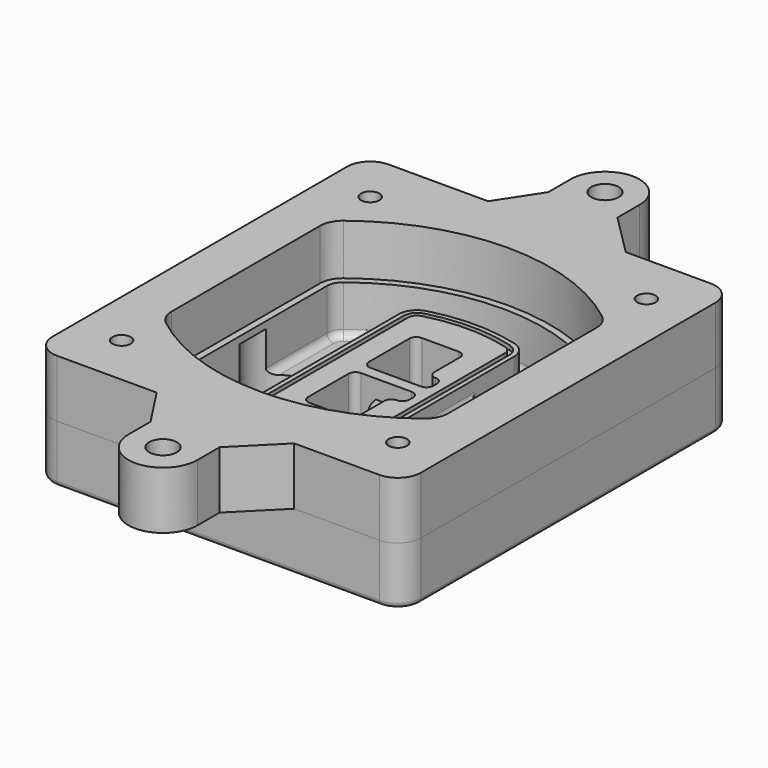
from build123d import *

# Parameters (mm, degrees)
F0_R      = 4
F1_DEPTH  = 25
F2_DEPTH  = 3
F3_DEPTH  = 18
F5_DEPTH  = 21
F6_DEPTH  = 2
F8_DEPTH  = 20
F9_DEPTH  = 16
F10_DEPTH = 25
F7_R      = 6
F7_R_2    = 4
F11_DEPTH = 6
F13_DEPTH = 9
F14_R     = 3
F15_R     = 2
F16_R     = 4
F16_R_2   = 6
F17_DEPTH = 25
F18_DEPTH = 25


# Not quite as in the source:
# - a feature names something its author has since deleted; it is built from what else it names


with BuildPart() as f1:
    # F0 (on Top) → F1 (new body)
    with BuildSketch(Plane.XY):
        with BuildLine():
            ThreePointArc((-80, -80), (-77.0710678119, -87.0710678119), (-70, -90))
            Line((-70, -90), (70, -90))
            ThreePointArc((70, -90), (77.0710678119, -87.0710678119), (80, -80))
            Line((80, -80), (80, 80))
            ThreePointArc((80, 80), (77.0710678119, 87.0710678119), (70, 90))
            Line((70, 90), (-70, 90))
            ThreePointArc((-70, 90), (-77.0710678119, 87.0710678119), (-80, 80))
            Line((-80, 80), (-80, -80))
        make_face()
        with Locations((-60, -67.5)):
            Circle(F0_R, mode=Mode.SUBTRACT)
        with Locations((60, -67.5)):
            Circle(F0_R, mode=Mode.SUBTRACT)
        with Locations((-60, 67.5)):
            Circle(F0_R, mode=Mode.SUBTRACT)
        with BuildLine():
            ThreePointArc((-64, 40.2934422872), (-62.5820384798, 46.4328484224), (-58.6153846154, 51.3286200352))
            ThreePointArc((-58.6153846154, 51.3286200352), (0, 71.5), (58.6153846154, 51.3286200352))
            ThreePointArc((58.6153846154, 51.3286200352), (62.5820384798, 46.4328484224), (64, 40.2934422872))
            Line((64, 40.2934422872), (64, -40.2934422872))
            ThreePointArc((64, -40.2934422872), (62.5820384798, -46.4328484224), (58.6153846154, -51.3286200352))
            ThreePointArc((58.6153846154, -51.3286200352), (0, -71.5), (-58.6153846154, -51.3286200352))
            ThreePointArc((-58.6153846154, -51.3286200352), (-62.5820384798, -46.4328484224), (-64, -40.2934422872))
            Line((-64, -40.2934422872), (-64, 40.2934422872))
        make_face(mode=Mode.SUBTRACT)
        with Locations((60, 67.5)):
            Circle(F0_R, mode=Mode.SUBTRACT)
        with BuildLine():
            ThreePointArc((58.6153846154, 51.3286200352), (0, 71.5), (-58.6153846154, 51.3286200352))
            ThreePointArc((-58.6153846154, 51.3286200352), (-62.5820384798, 46.4328484224), (-64, 40.2934422872))
            Line((-64, 40.2934422872), (-64, -40.2934422872))
            ThreePointArc((-64, -40.2934422872), (-62.5820384798, -46.4328484224), (-58.6153846154, -51.3286200352))
            ThreePointArc((-58.6153846154, -51.3286200352), (0, -71.5), (58.6153846154, -51.3286200352))
            ThreePointArc((58.6153846154, -51.3286200352), (62.5820384798, -46.4328484224), (64, -40.2934422872))
            Line((64, -40.2934422872), (64, 40.2934422872))
            ThreePointArc((64, 40.2934422872), (62.5820384798, 46.4328484224), (58.6153846154, 51.3286200352))
        make_face()
        with BuildLine():
            Line((-60, -40.2934422872), (-60, 40.2934422872))
            ThreePointArc((-60, 40.2934422872), (-58.9871703427, 44.6787323838), (-56.1538461538, 48.1757121072))
            ThreePointArc((-56.1538461538, 48.1757121072), (0, 67.5), (56.1538461538, 48.1757121072))
            ThreePointArc((56.1538461538, 48.1757121072), (58.9871703427, 44.6787323838), (60, 40.2934422872))
            Line((60, 40.2934422872), (60, -40.2934422872))
            ThreePointArc((60, -40.2934422872), (58.9871703427, -44.6787323838), (56.1538461538, -48.1757121072))
            ThreePointArc((56.1538461538, -48.1757121072), (0, -67.5), (-56.1538461538, -48.1757121072))
            ThreePointArc((-56.1538461538, -48.1757121072), (-58.9871703427, -44.6787323838), (-60, -40.2934422872))
        make_face(mode=Mode.SUBTRACT)
        with BuildLine():
            ThreePointArc((-56.1538461538, 48.1757121072), (-58.9871703427, 44.6787323838), (-60, 40.2934422872))
            Line((-60, 40.2934422872), (-60, -40.2934422872))
            ThreePointArc((-60, -40.2934422872), (-58.9871703427, -44.6787323838), (-56.1538461538, -48.1757121072))
            ThreePointArc((-56.1538461538, -48.1757121072), (0, -67.5), (56.1538461538, -48.1757121072))
            ThreePointArc((56.1538461538, -48.1757121072), (58.9871703427, -44.6787323838), (60, -40.2934422872))
            Line((60, -40.2934422872), (60, 40.2934422872))
            ThreePointArc((60, 40.2934422872), (58.9871703427, 44.6787323838), (56.1538461538, 48.1757121072))
            ThreePointArc((56.1538461538, 48.1757121072), (0, 67.5), (-56.1538461538, 48.1757121072))
        make_face()
        with BuildLine():
            ThreePointArc((54.3076923077, 45.8110311612), (56.2910192399, 43.3631453548), (57, 40.2934422872))
            Line((57, 40.2934422872), (57, -40.2934422872))
            ThreePointArc((57, -40.2934422872), (56.2910192399, -43.3631453548), (54.3076923077, -45.8110311612))
            ThreePointArc((54.3076923077, -45.8110311612), (0, -64.5), (-54.3076923077, -45.8110311612))
            ThreePointArc((-54.3076923077, -45.8110311612), (-56.2910192399, -43.3631453548), (-57, -40.2934422872))
            Line((-57, -40.2934422872), (-57, 40.2934422872))
            ThreePointArc((-57, 40.2934422872), (-56.2910192399, 43.3631453548), (-54.3076923077, 45.8110311612))
            ThreePointArc((-54.3076923077, 45.8110311612), (0, 64.5), (54.3076923077, 45.8110311612))
        make_face(mode=Mode.SUBTRACT)
        with BuildLine():
            Line((57, -40.2934422872), (57, 40.2934422872))
            ThreePointArc((57, 40.2934422872), (56.2910192399, 43.3631453548), (54.3076923077, 45.8110311612))
            ThreePointArc((54.3076923077, 45.8110311612), (0, 64.5), (-54.3076923077, 45.8110311612))
            ThreePointArc((-54.3076923077, 45.8110311612), (-56.2910192399, 43.3631453548), (-57, 40.2934422872))
            Line((-57, 40.2934422872), (-57, -40.2934422872))
            ThreePointArc((-57, -40.2934422872), (-56.2910192399, -43.3631453548), (-54.3076923077, -45.8110311612))
            ThreePointArc((-54.3076923077, -45.8110311612), (0, -64.5), (54.3076923077, -45.8110311612))
            ThreePointArc((54.3076923077, -45.8110311612), (56.2910192399, -43.3631453548), (57, -40.2934422872))
        make_face()
    extrude(amount=-F1_DEPTH)

    # F0 (on Top) → F2 (join)
    with BuildSketch(Plane.XY):
        with BuildLine():
            ThreePointArc((-56.1538461538, 48.1757121072), (-58.9871703427, 44.6787323838), (-60, 40.2934422872))
            Line((-60, 40.2934422872), (-60, -40.2934422872))
            ThreePointArc((-60, -40.2934422872), (-58.9871703427, -44.6787323838), (-56.1538461538, -48.1757121072))
            ThreePointArc((-56.1538461538, -48.1757121072), (0, -67.5), (56.1538461538, -48.1757121072))
            ThreePointArc((56.1538461538, -48.1757121072), (58.9871703427, -44.6787323838), (60, -40.2934422872))
            Line((60, -40.2934422872), (60, 40.2934422872))
            ThreePointArc((60, 40.2934422872), (58.9871703427, 44.6787323838), (56.1538461538, 48.1757121072))
            ThreePointArc((56.1538461538, 48.1757121072), (0, 67.5), (-56.1538461538, 48.1757121072))
        make_face()
        with BuildLine():
            ThreePointArc((54.3076923077, 45.8110311612), (56.2910192399, 43.3631453548), (57, 40.2934422872))
            Line((57, 40.2934422872), (57, -40.2934422872))
            ThreePointArc((57, -40.2934422872), (56.2910192399, -43.3631453548), (54.3076923077, -45.8110311612))
            ThreePointArc((54.3076923077, -45.8110311612), (0, -64.5), (-54.3076923077, -45.8110311612))
            ThreePointArc((-54.3076923077, -45.8110311612), (-56.2910192399, -43.3631453548), (-57, -40.2934422872))
            Line((-57, -40.2934422872), (-57, 40.2934422872))
            ThreePointArc((-57, 40.2934422872), (-56.2910192399, 43.3631453548), (-54.3076923077, 45.8110311612))
            ThreePointArc((-54.3076923077, 45.8110311612), (0, 64.5), (54.3076923077, 45.8110311612))
        make_face(mode=Mode.SUBTRACT)
    extrude(amount=F2_DEPTH)

    # F0 (on Top) → F3 (cut)
    with BuildSketch(Plane.XY):
        with BuildLine():
            Line((57, -40.2934422872), (57, 40.2934422872))
            ThreePointArc((57, 40.2934422872), (56.2910192399, 43.3631453548), (54.3076923077, 45.8110311612))
            ThreePointArc((54.3076923077, 45.8110311612), (0, 64.5), (-54.3076923077, 45.8110311612))
            ThreePointArc((-54.3076923077, 45.8110311612), (-56.2910192399, 43.3631453548), (-57, 40.2934422872))
            Line((-57, 40.2934422872), (-57, -40.2934422872))
            ThreePointArc((-57, -40.2934422872), (-56.2910192399, -43.3631453548), (-54.3076923077, -45.8110311612))
            ThreePointArc((-54.3076923077, -45.8110311612), (0, -64.5), (54.3076923077, -45.8110311612))
            ThreePointArc((54.3076923077, -45.8110311612), (56.2910192399, -43.3631453548), (57, -40.2934422872))
        make_face()
    extrude(amount=-F3_DEPTH, mode=Mode.SUBTRACT)

    # F4 (on face) → F5 (join, through all)
    with BuildSketch(Plane.XY.offset(3)):
        with BuildLine():
            ThreePointArc((-25, -39.2465276821), (-23.3511545998, -44.1109737193), (-19.0842911877, -46.9702398883))
            ThreePointArc((-19.0842911877, -46.9702398883), (0, -49.5), (19.0842911877, -46.9702398883))
            ThreePointArc((19.0842911877, -46.9702398883), (23.3511545998, -44.1109737193), (25, -39.2465276821))
            Line((25, -39.2465276821), (25, 39.2465276821))
            ThreePointArc((25, 39.2465276821), (23.3511545998, 44.1109737193), (19.0842911877, 46.9702398883))
            ThreePointArc((19.0842911877, 46.9702398883), (0, 49.5), (-19.0842911877, 46.9702398883))
            ThreePointArc((-19.0842911877, 46.9702398883), (-23.3511545998, 44.1109737193), (-25, 39.2465276821))
            Line((-25, 39.2465276821), (-25, -39.2465276821))
        make_face()
        with BuildLine():
            ThreePointArc((18.5632183908, 45.0393118368), (21.7633659499, 42.89486221), (23, 39.2465276821))
            Line((23, 39.2465276821), (23, -39.2465276821))
            ThreePointArc((23, -39.2465276821), (21.7633659499, -42.89486221), (18.5632183908, -45.0393118368))
            ThreePointArc((18.5632183908, -45.0393118368), (0, -47.5), (-18.5632183908, -45.0393118368))
            ThreePointArc((-18.5632183908, -45.0393118368), (-21.7633659499, -42.89486221), (-23, -39.2465276821))
            Line((-23, -39.2465276821), (-23, 39.2465276821))
            ThreePointArc((-23, 39.2465276821), (-21.7633659499, 42.89486221), (-18.5632183908, 45.0393118368))
            ThreePointArc((-18.5632183908, 45.0393118368), (0, 47.5), (18.5632183908, 45.0393118368))
        make_face(mode=Mode.SUBTRACT)
        with BuildLine():
            Line((23, -39.2465276821), (23, 39.2465276821))
            ThreePointArc((23, 39.2465276821), (21.7633659499, 42.89486221), (18.5632183908, 45.0393118368))
            ThreePointArc((18.5632183908, 45.0393118368), (0, 47.5), (-18.5632183908, 45.0393118368))
            ThreePointArc((-18.5632183908, 45.0393118368), (-21.7633659499, 42.89486221), (-23, 39.2465276821))
            Line((-23, 39.2465276821), (-23, -39.2465276821))
            ThreePointArc((-23, -39.2465276821), (-21.7633659499, -42.89486221), (-18.5632183908, -45.0393118368))
            ThreePointArc((-18.5632183908, -45.0393118368), (0, -47.5), (18.5632183908, -45.0393118368))
            ThreePointArc((18.5632183908, -45.0393118368), (21.7633659499, -42.89486221), (23, -39.2465276821))
        make_face()
        with BuildLine():
            ThreePointArc((18.0421455939, 43.1083837852), (20.1755772999, 41.6787507007), (21, 39.2465276821))
            Line((21, 39.2465276821), (21, -39.2465276821))
            ThreePointArc((21, -39.2465276821), (20.1755772999, -41.6787507007), (18.0421455939, -43.1083837852))
            ThreePointArc((18.0421455939, -43.1083837852), (0, -45.5), (-18.0421455939, -43.1083837852))
            ThreePointArc((-18.0421455939, -43.1083837852), (-20.1755772999, -41.6787507007), (-21, -39.2465276821))
            Line((-21, -39.2465276821), (-21, 39.2465276821))
            ThreePointArc((-21, 39.2465276821), (-20.1755772999, 41.6787507007), (-18.0421455939, 43.1083837852))
            ThreePointArc((-18.0421455939, 43.1083837852), (0, 45.5), (18.0421455939, 43.1083837852))
        make_face(mode=Mode.SUBTRACT)
        with BuildLine():
            Line((21, -39.2465276821), (21, 39.2465276821))
            ThreePointArc((21, 39.2465276821), (20.1755772999, 41.6787507007), (18.0421455939, 43.1083837852))
            ThreePointArc((18.0421455939, 43.1083837852), (0, 45.5), (-18.0421455939, 43.1083837852))
            ThreePointArc((-18.0421455939, 43.1083837852), (-20.1755772999, 41.6787507007), (-21, 39.2465276821))
            Line((-21, 39.2465276821), (-21, -39.2465276821))
            ThreePointArc((-21, -39.2465276821), (-20.1755772999, -41.6787507007), (-18.0421455939, -43.1083837852))
            ThreePointArc((-18.0421455939, -43.1083837852), (0, -45.5), (18.0421455939, -43.1083837852))
            ThreePointArc((18.0421455939, -43.1083837852), (20.1755772999, -41.6787507007), (21, -39.2465276821))
        make_face()
        with BuildLine():
            Line((-8, -2.5), (14, -2.5))
            ThreePointArc((14, -2.5), (16.1213203436, -3.3786796564), (17, -5.5))
            Line((17, -5.5), (17, -7.5))
            ThreePointArc((17, -7.5), (16.1213203436, -9.6213203436), (14, -10.5))
            ThreePointArc((14, -10.5), (11.8786796564, -11.3786796564), (11, -13.5))
            Line((11, -13.5), (11, -27.5))
            ThreePointArc((11, -27.5), (10.1213203436, -29.6213203436), (8, -30.5))
            Line((8, -30.5), (-8, -30.5))
            ThreePointArc((-8, -30.5), (-10.1213203436, -29.6213203436), (-11, -27.5))
            Line((-11, -27.5), (-11, -5.5))
            ThreePointArc((-11, -5.5), (-10.1213203436, -3.3786796564), (-8, -2.5))
        make_face(mode=Mode.SUBTRACT)
        with BuildLine():
            ThreePointArc((-8, 2.5), (-10.1213203436, 3.3786796564), (-11, 5.5))
            Line((-11, 5.5), (-11, 27.5))
            ThreePointArc((-11, 27.5), (-10.1213203436, 29.6213203436), (-8, 30.5))
            Line((-8, 30.5), (8, 30.5))
            ThreePointArc((8, 30.5), (10.1213203436, 29.6213203436), (11, 27.5))
            Line((11, 27.5), (11, 13.5))
            ThreePointArc((11, 13.5), (11.8786796564, 11.3786796564), (14, 10.5))
            ThreePointArc((14, 10.5), (16.1213203436, 9.6213203436), (17, 7.5))
            Line((17, 7.5), (17, 5.5))
            ThreePointArc((17, 5.5), (16.1213203436, 3.3786796564), (14, 2.5))
            Line((14, 2.5), (-8, 2.5))
        make_face(mode=Mode.SUBTRACT)
    extrude(amount=-F5_DEPTH)

    # F4 (on face) → F6 (cut)
    with BuildSketch(Plane.XY.offset(3)):
        with BuildLine():
            Line((23, -39.2465276821), (23, 39.2465276821))
            ThreePointArc((23, 39.2465276821), (21.7633659499, 42.89486221), (18.5632183908, 45.0393118368))
            ThreePointArc((18.5632183908, 45.0393118368), (0, 47.5), (-18.5632183908, 45.0393118368))
            ThreePointArc((-18.5632183908, 45.0393118368), (-21.7633659499, 42.89486221), (-23, 39.2465276821))
            Line((-23, 39.2465276821), (-23, -39.2465276821))
            ThreePointArc((-23, -39.2465276821), (-21.7633659499, -42.89486221), (-18.5632183908, -45.0393118368))
            ThreePointArc((-18.5632183908, -45.0393118368), (0, -47.5), (18.5632183908, -45.0393118368))
            ThreePointArc((18.5632183908, -45.0393118368), (21.7633659499, -42.89486221), (23, -39.2465276821))
        make_face()
        with BuildLine():
            ThreePointArc((18.0421455939, 43.1083837852), (20.1755772999, 41.6787507007), (21, 39.2465276821))
            Line((21, 39.2465276821), (21, -39.2465276821))
            ThreePointArc((21, -39.2465276821), (20.1755772999, -41.6787507007), (18.0421455939, -43.1083837852))
            ThreePointArc((18.0421455939, -43.1083837852), (0, -45.5), (-18.0421455939, -43.1083837852))
            ThreePointArc((-18.0421455939, -43.1083837852), (-20.1755772999, -41.6787507007), (-21, -39.2465276821))
            Line((-21, -39.2465276821), (-21, 39.2465276821))
            ThreePointArc((-21, 39.2465276821), (-20.1755772999, 41.6787507007), (-18.0421455939, 43.1083837852))
            ThreePointArc((-18.0421455939, 43.1083837852), (0, 45.5), (18.0421455939, 43.1083837852))
        make_face(mode=Mode.SUBTRACT)
    extrude(amount=-F6_DEPTH, mode=Mode.SUBTRACT)

    # F7 (on face) → F8 (join)
    with BuildSketch(Plane(origin=(0, 0, -25), x_dir=(1, 0, 0), z_dir=(0, 0, -1))):
        with BuildLine():
            ThreePointArc((3.28842436, 0), (16.7567035675, 13.4682792075), (30.224982775, 0))
            Line((30.224982775, 0), (35.224982775, 0))
            ThreePointArc((35.224982775, 0), (16.7567035675, 18.4682792075), (-1.71157564, 0))
            Line((-1.71157564, 0), (3.28842436, 0))
        make_face()
        with BuildLine():
            Line((3.28842436, 0), (30.224982775, 0))
            ThreePointArc((30.224982775, 0), (16.7567035675, 13.4682792075), (3.28842436, 0))
        make_face()
        with BuildLine():
            ThreePointArc((3.28842436, 0), (16.7567035675, -13.4682792075), (30.224982775, 0))
            Line((30.224982775, 0), (3.28842436, 0))
        make_face()
        with BuildLine():
            Line((35.224982775, 0), (30.224982775, 0))
            ThreePointArc((30.224982775, 0), (16.7567035675, -13.4682792075), (3.28842436, 0))
            Line((3.28842436, 0), (-1.71157564, 0))
            ThreePointArc((-1.71157564, 0), (16.7567035675, -18.4682792075), (35.224982775, 0))
        make_face()
    extrude(amount=-F8_DEPTH)

    # F7 (on face) → F9 (cut)
    with BuildSketch(Plane(origin=(0, 0, -25), x_dir=(1, 0, 0), z_dir=(0, 0, -1))):
        with BuildLine():
            Line((3.28842436, 0), (30.224982775, 0))
            ThreePointArc((30.224982775, 0), (16.7567035675, 13.4682792075), (3.28842436, 0))
        make_face()
        with BuildLine():
            ThreePointArc((3.28842436, 0), (16.7567035675, -13.4682792075), (30.224982775, 0))
            Line((30.224982775, 0), (3.28842436, 0))
        make_face()
    extrude(amount=-F9_DEPTH, mode=Mode.SUBTRACT)

    # F7 (on face) → F10 (cut)
    with BuildSketch(Plane(origin=(0, 0, -25), x_dir=(1, 0, 0), z_dir=(0, 0, -1))):
        with BuildLine():
            Line((-59.0318229325, 0), (-32.0952645175, 0))
            ThreePointArc((-32.0952645175, 0), (-45.563543725, 13.4682792075), (-59.0318229325, 0))
        make_face()
        with BuildLine():
            ThreePointArc((-59.0318229325, 0), (-45.563543725, -13.4682792075), (-32.0952645175, 0))
            Line((-32.0952645175, 0), (-59.0318229325, 0))
        make_face()
    extrude(amount=-F10_DEPTH, mode=Mode.SUBTRACT)

    # F7 (on face) → F11 (cut)
    with BuildSketch(Plane(origin=(0, 0, -25), x_dir=(1, 0, 0), z_dir=(0, 0, -1))):
        with Locations((60, -67.5)):
            Circle(F7_R)
        with Locations((60, -67.5)):
            Circle(F7_R_2, mode=Mode.SUBTRACT)
        with Locations((-60, -67.5)):
            Circle(F7_R)
        with Locations((-60, -67.5)):
            Circle(F7_R_2, mode=Mode.SUBTRACT)
        with Locations((-60, 67.5)):
            Circle(F7_R)
        with Locations((-60, 67.5)):
            Circle(F7_R_2, mode=Mode.SUBTRACT)
        with Locations((60, 67.5)):
            Circle(F7_R)
        with Locations((60, 67.5)):
            Circle(F7_R_2, mode=Mode.SUBTRACT)
    extrude(amount=-F11_DEPTH, mode=Mode.SUBTRACT)

    # F12 (on face) → F13 (cut, through all)
    with BuildSketch(Plane(origin=(0, 0, -9), x_dir=(1, 0, 0), z_dir=(0, 0, -1))):
        with BuildLine():
            Line((11, 13.5), (11, 17.5481537753))
            ThreePointArc((11, 17.5481537753), (2.5696536419, 11.8239143813), (-1.5415842455, 2.5))
            Line((-1.5415842455, 2.5), (3.5224848595, 2.5))
            ThreePointArc((3.5224848595, 2.5), (6.1857188154, 8.3455872281), (11.2536447004, 12.2927168648))
            ThreePointArc((11.2536447004, 12.2927168648), (11.0640958889, 12.8831798879), (11, 13.5))
        make_face()
        with BuildLine():
            ThreePointArc((11.2536447004, -12.2927168648), (6.1857188154, -8.3455872281), (3.5224848595, -2.5))
            Line((3.5224848595, -2.5), (-1.5415842455, -2.5))
            ThreePointArc((-1.5415842455, -2.5), (2.5696536419, -11.8239143813), (11, -17.5481537753))
            Line((11, -17.5481537753), (11, -13.5))
            ThreePointArc((11, -13.5), (11.0640958889, -12.8831798879), (11.2536447004, -12.2927168648))
        make_face()
        with BuildLine():
            ThreePointArc((11.2536447004, 12.2927168648), (6.1857188154, 8.3455872281), (3.5224848595, 2.5))
            Line((3.5224848595, 2.5), (14, 2.5))
            ThreePointArc((14, 2.5), (16.1213203436, 3.3786796564), (17, 5.5))
            Line((17, 5.5), (17, 7.5))
            ThreePointArc((17, 7.5), (16.1213203436, 9.6213203436), (14, 10.5))
            ThreePointArc((14, 10.5), (12.3601599782, 10.9878446101), (11.2536447004, 12.2927168648))
        make_face()
        with BuildLine():
            Line((14, -2.5), (3.5224848595, -2.5))
            ThreePointArc((3.5224848595, -2.5), (6.1857188154, -8.3455872281), (11.2536447004, -12.2927168648))
            ThreePointArc((11.2536447004, -12.2927168648), (12.3601599782, -10.9878446101), (14, -10.5))
            ThreePointArc((14, -10.5), (16.1213203436, -9.6213203436), (17, -7.5))
            Line((17, -7.5), (17, -5.5))
            ThreePointArc((17, -5.5), (16.1213203436, -3.3786796564), (14, -2.5))
        make_face()
    extrude(amount=F13_DEPTH, mode=Mode.SUBTRACT)

    # F14
    f14_edges = [f1.edges().sort_by_distance(p)[0] for p in [
        (-57, -23.703476, -18),
        (-57, 23.703476, -18),
        (25, 0, -5),
        (25, 16.526506, -11.5),
        (25, -16.526506, -11.5),
        (25, -27.886517, -18),
        (35.224983, 0, -18),
    ]]
    fillet(f14_edges, radius=F14_R)

    # F15
    f15_edges = [f1.edges().sort_by_distance(p)[0] for p in [
        (0, -90, -25),
    ]]
    fillet(f15_edges, radius=F15_R)


with BuildPart() as f17:
    # F16 (on face) → F17 (new body)
    with BuildSketch(Plane.XY):
        with BuildLine():
            Line((-26.7517124091, 90), (-70, 90))
            ThreePointArc((-70, 90), (-77.0710678119, 87.0710678119), (-80, 80))
            Line((-80, 80), (-80, -80))
            ThreePointArc((-80, -80), (-77.0710678119, -87.0710678119), (-70, -90))
            Line((-70, -90), (-26.7517124091, -90))
            Line((-26.7517124091, -90), (33, -90))
            Line((33, -90), (70, -90))
            ThreePointArc((70, -90), (77.0710678119, -87.0710678119), (80, -80))
            Line((80, -80), (80, 80))
            ThreePointArc((80, 80), (77.0710678119, 87.0710678119), (70, 90))
            Line((70, 90), (33, 90))
            Line((33, 90), (-26.7517124091, 90))
        make_face()
        with Locations((-60, -67.5)):
            Circle(F16_R, mode=Mode.SUBTRACT)
        with Locations((60, -67.5)):
            Circle(F16_R, mode=Mode.SUBTRACT)
        with Locations((-60, 67.5)):
            Circle(F16_R, mode=Mode.SUBTRACT)
        with BuildLine():
            ThreePointArc((-56.1538461538, 48.1757121072), (0, 67.5), (56.1538461538, 48.1757121072))
            ThreePointArc((56.1538461538, 48.1757121072), (58.9871703427, 44.6787323838), (60, 40.2934422872))
            Line((60, 40.2934422872), (60, -40.2934422872))
            ThreePointArc((60, -40.2934422872), (58.9871703427, -44.6787323838), (56.1538461538, -48.1757121072))
            ThreePointArc((56.1538461538, -48.1757121072), (0, -67.5), (-56.1538461538, -48.1757121072))
            ThreePointArc((-56.1538461538, -48.1757121072), (-58.9871703427, -44.6787323838), (-60, -40.2934422872))
            Line((-60, -40.2934422872), (-60, 40.2934422872))
            ThreePointArc((-60, 40.2934422872), (-58.9871703427, 44.6787323838), (-56.1538461538, 48.1757121072))
        make_face(mode=Mode.SUBTRACT)
        with Locations((60, 67.5)):
            Circle(F16_R, mode=Mode.SUBTRACT)
        with BuildLine():
            Line((-15, 108), (-26.7517124091, 90))
            Line((-26.7517124091, 90), (33, 90))
            Line((33, 90), (15, 108))
            Line((15, 108), (15, 120))
            ThreePointArc((15, 120), (0, 135), (-15, 120))
            Line((-15, 120), (-15, 108))
        make_face()
        with Locations((0, 120)):
            Circle(F16_R_2, mode=Mode.SUBTRACT)
        with BuildLine():
            Line((33, -90), (-26.7517124091, -90))
            Line((-26.7517124091, -90), (-15, -108))
            Line((-15, -108), (-15, -120))
            ThreePointArc((-15, -120), (0, -135), (15, -120))
            Line((15, -120), (15, -108))
            Line((15, -108), (33, -90))
        make_face()
        with Locations((0, -120)):
            Circle(F16_R_2, mode=Mode.SUBTRACT)
    extrude(amount=F17_DEPTH)


with BuildPart() as f18:
    # F16 (on face) → F18 (new body)
    with BuildSketch(Plane.XY):
        with BuildLine():
            Line((-26.7517124091, 90), (-70, 90))
            ThreePointArc((-70, 90), (-77.0710678119, 87.0710678119), (-80, 80))
            Line((-80, 80), (-80, -80))
            ThreePointArc((-80, -80), (-77.0710678119, -87.0710678119), (-70, -90))
            Line((-70, -90), (-26.7517124091, -90))
            Line((-26.7517124091, -90), (33, -90))
            Line((33, -90), (70, -90))
            ThreePointArc((70, -90), (77.0710678119, -87.0710678119), (80, -80))
            Line((80, -80), (80, 80))
            ThreePointArc((80, 80), (77.0710678119, 87.0710678119), (70, 90))
            Line((70, 90), (33, 90))
            Line((33, 90), (-26.7517124091, 90))
        make_face()
        with Locations((-60, -67.5)):
            Circle(F16_R, mode=Mode.SUBTRACT)
        with Locations((60, -67.5)):
            Circle(F16_R, mode=Mode.SUBTRACT)
        with Locations((-60, 67.5)):
            Circle(F16_R, mode=Mode.SUBTRACT)
        with BuildLine():
            ThreePointArc((-56.1538461538, 48.1757121072), (0, 67.5), (56.1538461538, 48.1757121072))
            ThreePointArc((56.1538461538, 48.1757121072), (58.9871703427, 44.6787323838), (60, 40.2934422872))
            Line((60, 40.2934422872), (60, -40.2934422872))
            ThreePointArc((60, -40.2934422872), (58.9871703427, -44.6787323838), (56.1538461538, -48.1757121072))
            ThreePointArc((56.1538461538, -48.1757121072), (0, -67.5), (-56.1538461538, -48.1757121072))
            ThreePointArc((-56.1538461538, -48.1757121072), (-58.9871703427, -44.6787323838), (-60, -40.2934422872))
            Line((-60, -40.2934422872), (-60, 40.2934422872))
            ThreePointArc((-60, 40.2934422872), (-58.9871703427, 44.6787323838), (-56.1538461538, 48.1757121072))
        make_face(mode=Mode.SUBTRACT)
        with Locations((60, 67.5)):
            Circle(F16_R, mode=Mode.SUBTRACT)
        with BuildLine():
            Line((-15, 108), (-26.7517124091, 90))
            Line((-26.7517124091, 90), (33, 90))
            Line((33, 90), (15, 108))
            Line((15, 108), (15, 120))
            ThreePointArc((15, 120), (0, 135), (-15, 120))
            Line((-15, 120), (-15, 108))
        make_face()
        with Locations((0, 120)):
            Circle(F16_R_2, mode=Mode.SUBTRACT)
        with BuildLine():
            Line((33, -90), (-26.7517124091, -90))
            Line((-26.7517124091, -90), (-15, -108))
            Line((-15, -108), (-15, -120))
            ThreePointArc((-15, -120), (0, -135), (15, -120))
            Line((15, -120), (15, -108))
            Line((15, -108), (33, -90))
        make_face()
        with Locations((0, -120)):
            Circle(F16_R_2, mode=Mode.SUBTRACT)
    extrude(amount=F18_DEPTH)


solid = Compound([f1.part, f17.part, f18.part])
